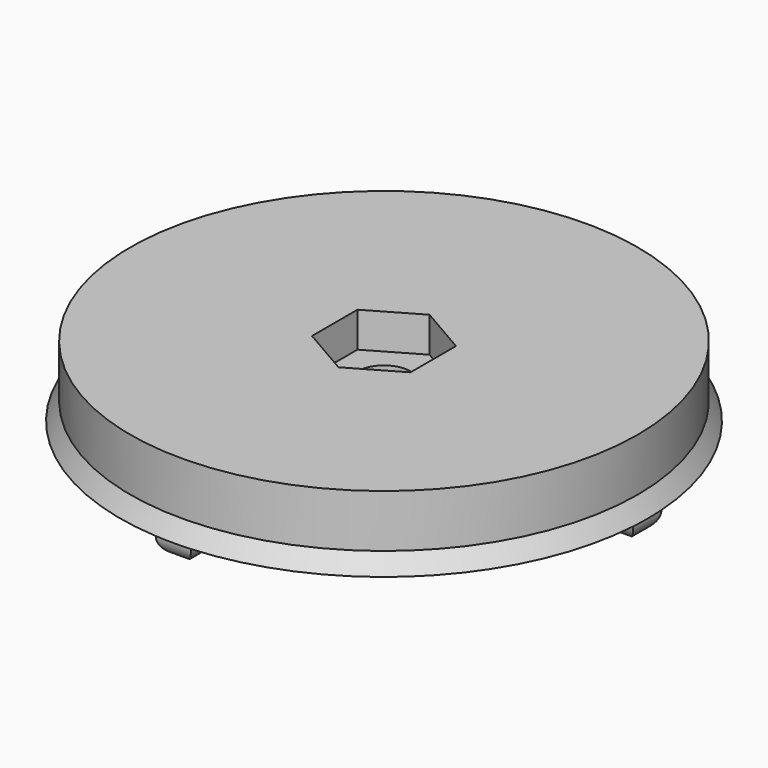
from build123d import *

# Parameters (mm, degrees)
F0_R     = 15
F1_DEPTH = 1
F1_TAPER = 30
F2_DEPTH = 3
F4_DEPTH = 2
F5_R     = 1.5
F6_DEPTH = 2.001
F7_W     = 13.4332590942
F7_H     = 2
F7_W_2   = 2
F7_H_2   = 13.4332590942
F8_DEPTH = 1
F9_R     = 0.99999


# Not quite as in the source:
# - a fillet or chamfer is up to 0.001 mm smaller than in the source, because OpenCascade refuses the exact size


with BuildPart() as f1:
    # F0 (on Top) → F1 (new body)
    with BuildSketch(Plane.XY):
        Circle(F0_R)
    extrude(amount=F1_DEPTH, taper=F1_TAPER)

    # F2 (add): a face of the model
    f2_faces = [f1.faces().sort_by_distance(p)[0] for p in [
        (0, 0, 1),
    ]]
    extrude(f2_faces, amount=F2_DEPTH)

    # F3 (on face) → F4 (cut)
    with BuildSketch(Plane.XY.offset(4)):
        Polygon((2.8, -1.6165807537), (2.8, 1.6165807537), (0, 3.2331615075), (-2.8, 1.6165807537), (-2.8, -1.6165807537), (0, -3.2331615075), align=None)
    extrude(amount=-F4_DEPTH, mode=Mode.SUBTRACT)

    # F5 (on face) → F6 (cut, through all)
    with BuildSketch(Plane.XY.offset(2)):
        Circle(F5_R)
    extrude(amount=-F6_DEPTH, mode=Mode.SUBTRACT)

    # F7 (on face) → F8 (join)
    with BuildSketch(Plane(origin=(0, 0, 0), x_dir=(1, 0, 0), z_dir=(0, 0, -1))):
        with Locations((-8.25, 0)):
            Rectangle(F7_W, F7_H)
        with Locations((0, 8.25)):
            Rectangle(F7_W_2, F7_H_2)
        with Locations((8.25, 0)):
            Rectangle(F7_W, F7_H)
        with Locations((0, -8.25)):
            Rectangle(F7_W_2, F7_H_2)
    extrude(amount=F8_DEPTH)

    # F9 (radius 1 in the source; OpenCascade refuses exactly that, so slightly less here)
    f9_edges = [f1.edges().sort_by_distance(p)[0] for p in [
        (-1, 8.25, -1),
        (1, 8.25, -1),
        (8.25, 1, -1),
        (14.96663, 0, -1),
        (8.25, -1, -1),
        (1.53337, 0, -1),
        (-8.25, 1, -1),
        (-8.25, -1, -1),
        (1, -8.25, -1),
        (-1, -8.25, -1),
        (0, 14.96663, -1),
        (0, 1.53337, -1),
        (0, -1.53337, -1),
        (-1.53337, 0, -1),
        (-14.96663, 0, -1),
        (0, -14.96663, -1),
    ]]
    fillet(f9_edges, radius=F9_R)


solid = f1.part
